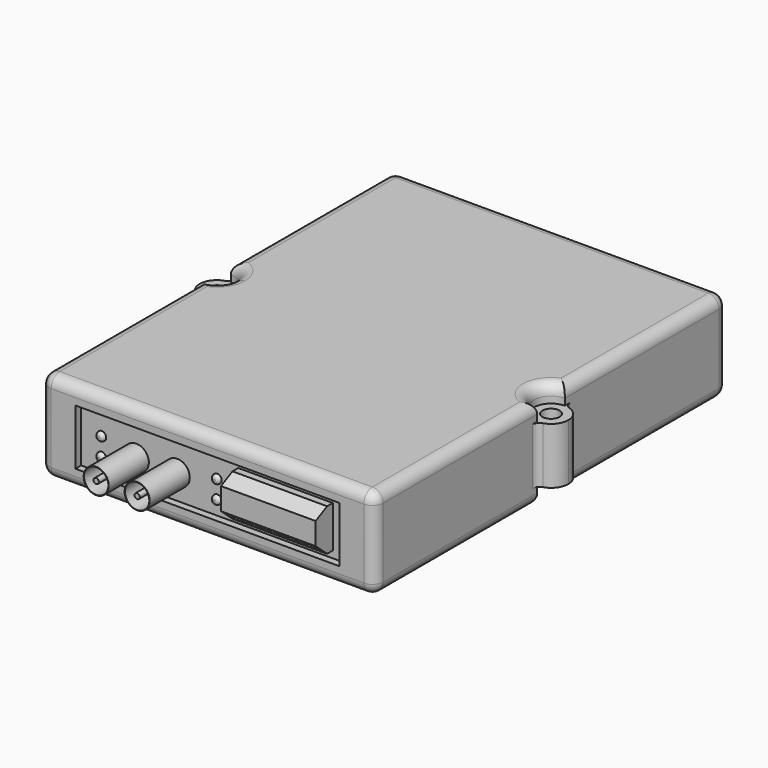
from build123d import *

# Parameters (mm, degrees)
F1_DEPTH  = 12.7
F2_DEPTH  = 7.862
F3_R      = 3
F4_R      = 2
F5_W      = 73.78
F5_H      = 15.55
F6_DEPTH  = 2
F7_W      = 73.78
F7_H      = 15.55
F8_DEPTH  = 2
F9_W      = 11.176
F9_H      = 11.938
F10_DEPTH = 5
F11_SIZE2 = 4
F11_SIZE  = 2
F12_SIZE2 = 4.5
F12_SIZE  = 3
F13_R     = 1.5
F14_DEPTH = 3
F15_W     = 26.416
F15_H     = 11.684
F16_DEPTH = 6
F17_SIZE2 = 4
F17_SIZE  = 2
F18_SIZE2 = 3.5
F18_SIZE  = 4
F19_W     = 3.8
F19_H     = 3.8
F20_DEPTH = 3
F21_W     = 3
F21_H     = 3
F22_DEPTH = 4
F9_R      = 1.5
F9_R_2    = 0.1520799932
F23_DEPTH = 6
F9_R_3    = 3.175
F24_DEPTH = 0.2
F25_R     = 3.5
F25_R_2   = 3.4
F25_R_3   = 0.75
F26_DEPTH = 14
F25_R_4   = 1.25
F28_DEPTH = 1
F29_R     = 0.99999


# Not quite as in the source:
# - a fillet or chamfer is up to 0.001 mm smaller than in the source, because OpenCascade refuses the exact size


with BuildPart() as f1:
    # F0 (on Top) → F1 (new body, symmetric)
    with BuildSketch(Plane.XY):
        with BuildLine():
            Line((-46.65, -61.6), (46.65, -61.6))
            Line((46.65, -61.6), (46.65, -4.826))
            ThreePointArc((46.65, -4.826), (41.824, 0), (46.65, 4.826))
            Line((46.65, 4.826), (46.65, 61.6))
            Line((46.65, 61.6), (-46.65, 61.6))
            Line((-46.65, 61.6), (-46.65, 4.826))
            ThreePointArc((-46.65, 4.826), (-43.237502674, 3.412497326), (-41.824, 0))
            ThreePointArc((-41.824, 0), (-43.237502674, -3.412497326), (-46.65, -4.826))
            Line((-46.65, -4.826), (-46.65, -61.6))
        make_face()
    extrude(amount=F1_DEPTH, both=True)

    # F0 (on Top) → F2 (join, symmetric)
    with BuildSketch(Plane.XY):
        with BuildLine():
            ThreePointArc((-46.65, 4.826), (-51.476, 0), (-46.65, -4.826))
            Line((-46.65, -4.826), (-46.65, -2.413))
            ThreePointArc((-46.65, -2.413), (-49.063, 0), (-46.65, 2.413))
            Line((-46.65, 2.413), (-46.65, 4.826))
        make_face()
        with BuildLine():
            Line((46.65, -2.413), (46.65, -4.826))
            ThreePointArc((46.65, -4.826), (50.062497326, -3.412497326), (51.476, 0))
            ThreePointArc((51.476, 0), (50.062497326, 3.412497326), (46.65, 4.826))
            Line((46.65, 4.826), (46.65, 2.413))
            ThreePointArc((46.65, 2.413), (48.356248663, 1.706248663), (49.063, 0))
            ThreePointArc((49.063, 0), (48.356248663, -1.706248663), (46.65, -2.413))
        make_face()
        with BuildLine():
            Line((-46.65, -2.413), (-46.65, -4.826))
            ThreePointArc((-46.65, -4.826), (-43.237502674, -3.412497326), (-41.824, 0))
            ThreePointArc((-41.824, 0), (-43.237502674, 3.412497326), (-46.65, 4.826))
            Line((-46.65, 4.826), (-46.65, 2.413))
            ThreePointArc((-46.65, 2.413), (-44.943751337, 1.706248663), (-44.237, 0))
            ThreePointArc((-44.237, 0), (-44.943751337, -1.706248663), (-46.65, -2.413))
        make_face()
        with BuildLine():
            ThreePointArc((46.65, 4.826), (41.824, 0), (46.65, -4.826))
            Line((46.65, -4.826), (46.65, -2.413))
            ThreePointArc((46.65, -2.413), (44.237, 0), (46.65, 2.413))
            Line((46.65, 2.413), (46.65, 4.826))
        make_face()
    extrude(amount=F2_DEPTH, both=True)

    # F3
    f3_edges = [f1.edges().sort_by_distance(p)[0] for p in [
        (-46.65, -33.213, 12.7),
        (0, -61.6, 12.7),
        (46.65, -33.213, 12.7),
        (41.824, 0, 12.7),
        (46.65, 33.213, 12.7),
        (0, 61.6, 12.7),
        (-46.65, 33.213, 12.7),
        (-41.824, 0, 12.7),
        (-46.65, -33.213, -12.7),
        (0, -61.6, -12.7),
        (46.65, -33.213, -12.7),
        (41.824, 0, -12.7),
        (46.65, 33.213, -12.7),
        (0, 61.6, -12.7),
        (-46.65, 33.213, -12.7),
        (-41.824, 0, -12.7),
        (46.65, -61.6, 0),
        (-46.65, -61.6, 0),
        (-46.65, 61.6, 0),
        (46.65, 61.6, 0),
    ]]
    fillet(f3_edges, radius=F3_R)

    # F4
    f4_edges = [f1.edges().sort_by_distance(p)[0] for p in [
        (-46.65, -4.826, 0),
        (-46.65, 4.826, 0),
        (46.65, -4.826, 0),
        (46.65, 4.826, 0),
    ]]
    fillet(f4_edges, radius=F4_R)

    # F5 (on face) → F6 (cut)
    with BuildSketch(Plane.XZ.offset(61.6)):
        Rectangle(F5_W, F5_H)
    extrude(amount=-F6_DEPTH, mode=Mode.SUBTRACT)

    # F7 (on face) → F8 (cut)
    with BuildSketch(Plane(origin=(0, 61.6, 0), x_dir=(-1, 0, 0), z_dir=(0, 1, 0))):
        Rectangle(F7_W, F7_H)
    extrude(amount=-F8_DEPTH, mode=Mode.SUBTRACT)

    # F9 (on face) → F23 (cut)
    with BuildSketch(Plane(origin=(0, 59.6, 0), x_dir=(-1, 0, 0), z_dir=(0, 1, 0))):
        with Locations((-27.746, 0)):
            Circle(F9_R)
        with Locations((-27.746, 0)):
            Circle(F9_R_2, mode=Mode.SUBTRACT)
    extrude(amount=-F23_DEPTH, mode=Mode.SUBTRACT)

    # F9 (on face) → F24 (join)
    with BuildSketch(Plane(origin=(0, 59.6, 0), x_dir=(-1, 0, 0), z_dir=(0, 1, 0))):
        with Locations((-27.746, 0)):
            Circle(F9_R_3)
        with Locations((-27.746, 0)):
            Circle(F9_R, mode=Mode.SUBTRACT)
    extrude(amount=F24_DEPTH)

    # F25 (on face) → F26 (join)
    with BuildSketch(Plane.XZ.offset(59.6)):
        with Locations((-10.058, -0.917)):
            Circle(F25_R)
        with Locations((-10.058, -0.917)):
            Circle(F25_R_2, mode=Mode.SUBTRACT)
        with Locations((-21.488, -0.917)):
            Circle(F25_R)
        with Locations((-21.488, -0.917)):
            Circle(F25_R_2, mode=Mode.SUBTRACT)
        with Locations((-21.488, -0.917)):
            Circle(F25_R_3)
        with Locations((-10.058, -0.917)):
            Circle(F25_R_3)
    extrude(amount=F26_DEPTH)

    # F25 (on face) → F28 (join)
    with BuildSketch(Plane.XZ.offset(59.6)):
        with Locations((1.118, -3.775)):
            Circle(F25_R_4)
        with Locations((1.118, 1.305)):
            Circle(F25_R_4)
        with Locations((-31.14, -3.775)):
            Circle(F25_R_4)
        with Locations((-31.14, 1.305)):
            Circle(F25_R_4)
    extrude(amount=F28_DEPTH)

    # F29 (radius 1 in the source; OpenCascade refuses exactly that, so slightly less here)
    f29_edges = [f1.edges().sort_by_distance(p)[0] for p in [
        (-32.39, -60.6, 1.305),
        (-32.39, -60.6, -3.775),
        (-0.132, -60.6, -3.775),
        (-0.132, -60.6, 1.305),
    ]]
    fillet(f29_edges, radius=F29_R)


with BuildPart() as f10:
    # F9 (on face) → F10 (new body)
    with BuildSketch(Plane(origin=(0, 59.6, 0), x_dir=(-1, 0, 0), z_dir=(0, 1, 0))):
        with Locations((-12.506, 0)):
            Rectangle(F9_W, F9_H)
    extrude(amount=F10_DEPTH)

    # F11
    f11_edges = [f10.edges().sort_by_distance(p)[0] for p in [
        (12.506, 64.6, 5.969),
    ]]
    f11_side = f10.faces().sort_by_distance((12.506, 64.6, 0))[0]
    chamfer(f11_edges, length=F11_SIZE, length2=F11_SIZE2, reference=f11_side)

    # F12
    f12_edges = [f10.edges().sort_by_distance(p)[0] for p in [
        (12.506, 64.6, -5.969),
    ]]
    f12_side = f10.faces().sort_by_distance((12.506, 62.1, -5.969))[0]
    chamfer(f12_edges, length=F12_SIZE, length2=F12_SIZE2, reference=f12_side)

    # F13 (on face) → F14 (cut)
    with BuildSketch(Plane.XY.offset(5.969)):
        with Locations((15.506, 62.9279017448)):
            Circle(F13_R)
        with Locations((9.506, 62.9279017448)):
            Circle(F13_R)
    extrude(amount=-F14_DEPTH, mode=Mode.SUBTRACT)

    # F19 (on face) → F20 (cut)
    with BuildSketch(Plane(origin=(0, 64.6, 0), x_dir=(-1, 0, 0), z_dir=(0, 1, 0))):
        with Locations((-15.506, -3.5991897196)):
            Rectangle(F19_W, F19_H)
        with Locations((-9.506, -3.5991897196)):
            Rectangle(F19_W, F19_H)
    extrude(amount=-F20_DEPTH, mode=Mode.SUBTRACT)


with BuildPart() as f16:
    # F15 (on face) → F16 (new body)
    with BuildSketch(Plane.XZ.offset(59.6)):
        with Locations((20.182, 0)):
            Rectangle(F15_W, F15_H)
    extrude(amount=F16_DEPTH)

    # F17
    f17_edges = [f16.edges().sort_by_distance(p)[0] for p in [
        (20.182, -65.6, 5.842),
    ]]
    f17_side = f16.faces().sort_by_distance((20.182, -65.6, 0))[0]
    chamfer(f17_edges, length=F17_SIZE, length2=F17_SIZE2, reference=f17_side)

    # F18
    f18_edges = [f16.edges().sort_by_distance(p)[0] for p in [
        (20.182, -65.6, -5.842),
    ]]
    f18_side = f16.faces().sort_by_distance((20.182, -62.6, -5.842))[0]
    chamfer(f18_edges, length=F18_SIZE, length2=F18_SIZE2, reference=f18_side)

    # F21 (on face) → F22 (cut)
    with BuildSketch(Plane.XZ.offset(65.6)):
        with Locations((10.022, -4.2285963558)):
            Rectangle(F21_W, F21_H)
        with Locations((15.102, -4.2285963558)):
            Rectangle(F21_W, F21_H)
        with Locations((20.182, -4.2285963558)):
            Rectangle(F21_W, F21_H)
        with Locations((25.262, -4.2285963558)):
            Rectangle(F21_W, F21_H)
        with Locations((30.342, -4.2285963558)):
            Rectangle(F21_W, F21_H)
    extrude(amount=-F22_DEPTH, mode=Mode.SUBTRACT)


solid = Compound([f1.part, f10.part, f16.part])
